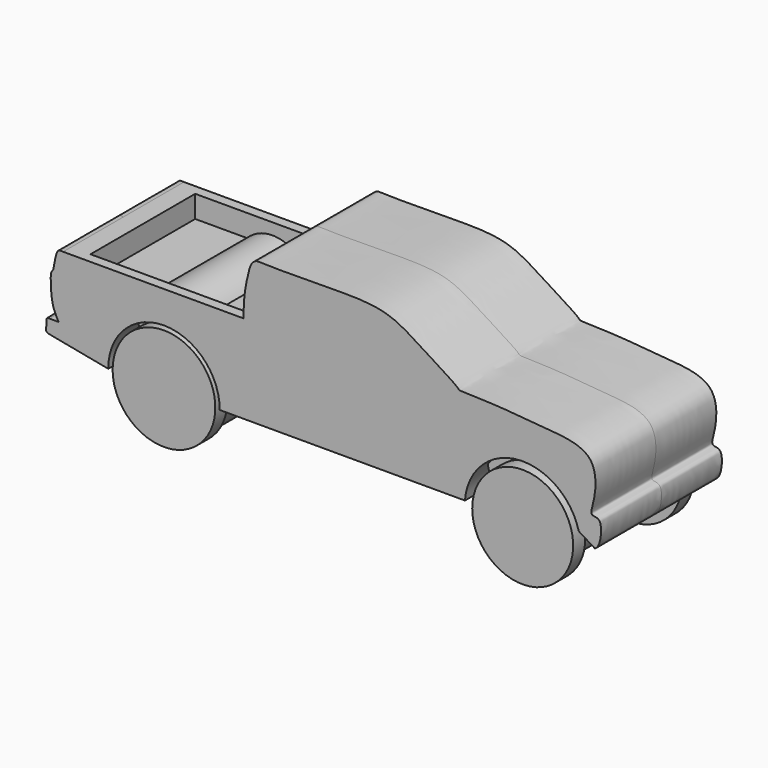
from build123d import *

# Parameters (mm, degrees)
F1_DEPTH  = 19.05
F2_W      = 40.64
F2_H      = 33.02
F3_DEPTH  = 5.588
F4_R      = 12.9540001242
F5_DEPTH  = 3.81
F4_R_2    = 12.7302206493
F9_R      = 9.0231683156
F10_DEPTH = 30.988
F11_R     = 11.353288786
F12_DEPTH = 30.988
F13_R     = 11.9558866418
F14_DEPTH = 32.258
F15_R     = 6.4554552036
F16_DEPTH = 30.734


with BuildPart() as f1:
    # F0 (on Front) → F1 (new body, symmetric)
    with BuildSketch(Plane.XZ):
        with BuildLine():
            add(Edge.make_bspline(
                [(-69.2842155695, -1.5603305073), (-69.5350025172, -1.5399307664), (-70.1964658552, -1.526121286), (-69.9018841173, -3.0286902092), (-70.3645967063, -4.8077768479), (-69.5958865333, -4.978686168), (-69.2788809538, -5.04994113)],
                knots=[0, 0, 0, 0, 0.1954252336, 0.4695328217, 0.7775236757, 1, 1, 1, 1], degree=3))
            Line((-69.2788809538, -5.04994113), (-54.4446744025, -7.8905327246))
            ThreePointArc((-54.4446744025, -7.8905327246), (-40.3995271772, 6.3133119394), (-26.354379952, -7.8905327246))
            Line((-26.354379952, -7.8905327246), (35.5073921382, -7.8905327246))
            ThreePointArc((35.5073921382, -7.8905327246), (48.7999211019, 5.5232241619), (64.2289370298, -5.3655621596))
            Line((64.2289370298, -5.3655621596), (68.332016468, -7.8905327246))
            add(Edge.make_bspline(
                [(68.332016468, -7.8905327246), (68.7067913051, -7.5679449616), (69.714492426, -6.7005653561), (70.3172984159, -0.4392585426), (66.7802927419, -1.0958089063), (68.4028013282, 2.9762612334), (69.2917253521, 14.2725497335), (53.5065140597, 14.7113305441), (43.8771565321, 16.0310681315), (33.8781446405, 15.9310273294), (33.9330328582, 16.6675611215), (26.0002542616, 21.5508658082), (18.2176068002, 26.7807544456), (11.4548434095, 28.1451041805), (3.6587892983, 28.3191044585), (-14.7558362833, 27.9741795524), (-17.1668552051, 28.3644164723), (-18.5859335818, 27.0949449022), (-19.2248198393, 24.36459907), (-20.2441867929, 19.8982618034), (-20.3211424661, 16.2882279072), (-20.3614756465, 14.3961757421)],
                knots=[0, 0, 0, 0, 0.0298592954, 0.0802861944, 0.110508584, 0.1504361757, 0.217563582, 0.2973555397, 0.3741757692, 0.438561904, 0.4519709004, 0.5165255825, 0.5881373031, 0.6432617714, 0.7085227769, 0.8031750452, 0.8361448558, 0.8632792375, 0.8998543586, 0.9475127428, 1, 1, 1, 1], degree=3))
            Line((-20.3614756465, 14.3961757421), (-65.8321008086, 14.3961757421))
            add(Edge.make_bspline(
                [(-65.8321008086, 14.3961757421), (-66.1119049823, 14.4054631172), (-66.6227405068, 14.4224189798), (-67.2879149417, 14.2751954831), (-67.9931529597, 11.9924706508), (-68.1930622811, 9.4607186493), (-69.0930767314, 9.0286087442), (-68.9238735496, 4.2425680846), (-68.3896505368, 1.0708895061), (-67.4304833389, -0.7146991208), (-66.9762343168, -1.5603305073)],
                knots=[0, 0, 0, 0, 0.0788218688, 0.1439042534, 0.2790854206, 0.4187108143, 0.4966559878, 0.6831908786, 0.8499633496, 1, 1, 1, 1], degree=3))
            Line((-66.9762343168, -1.5603305073), (-69.2842155695, -1.5603305073))
        make_face()
    extrude(amount=F1_DEPTH, both=True)

    # F2 (on face) → F3 (cut)
    with BuildSketch(Plane.XY.offset(14.3961757421)):
        with Locations((-40.6465960781, 0)):
            Rectangle(F2_W, F2_H)
    extrude(amount=-F3_DEPTH, mode=Mode.SUBTRACT)



with BuildPart() as f5:
    # F4 (on face) → F5 (new body)
    with BuildSketch(Plane(origin=(0, 19.05, 0), x_dir=(-1, 0, 0), z_dir=(0, 1, 0))):
        with Locations((40.3995271772, -7.7327218372)):
            Circle(F4_R)
    extrude(amount=-F5_DEPTH)


with BuildPart() as f5b:
    # F4 (on face) → F5, piece 2 (new body)
    with BuildSketch(Plane(origin=(0, 19.05, 0), x_dir=(-1, 0, 0), z_dir=(0, 1, 0))):
        with Locations((-50.0800661584, -9.0384282465)):
            Circle(F4_R_2)
    extrude(amount=-F5_DEPTH)


with BuildPart() as f6_1:
    # F6: instance of F5
    add(f5.part.mirror(Plane.XZ))


with BuildPart() as f6_2:
    # F6: instance of F5b
    add(f5b.part.mirror(Plane.XZ))


with BuildPart() as f1_1:
    add(f1.part)

    add(f5.part)  # F10 merges F5

    add(f6_1.part)  # F10 merges F6_1
    # F9 (on face) → F10 (join)
    with BuildSketch(Plane.XZ.offset(-15.24)):
        with Locations((-40.4575429857, 3.333261935)):
            Circle(F9_R)
    extrude(amount=F10_DEPTH)


    add(f5b.part)  # F12 merges F5b

    add(f6_2.part)  # F12 merges F6_2
    # F11 (on face) → F12 (join)
    with BuildSketch(Plane(origin=(0, -15.24, 0), x_dir=(-1, 0, 0), z_dir=(0, 1, 0))):
        with Locations((-49.4373105466, 1.3395160204)):
            Circle(F11_R)
    extrude(amount=F12_DEPTH)

    # F13 (on face) → F14 (join)
    with BuildSketch(Plane(origin=(0, -15.24, 0), x_dir=(-1, 0, 0), z_dir=(0, 1, 0))):
        with Locations((40.3995271772, -7.7327218372)):
            Circle(F13_R)
    extrude(amount=F14_DEPTH)

    # F15 (on face) → F16 (join)
    with BuildSketch(Plane(origin=(0, -15.24, 0), x_dir=(-1, 0, 0), z_dir=(0, 1, 0))):
        with Locations((-50.299461931, -13.3715048432)):
            Circle(F15_R)
    extrude(amount=F16_DEPTH)


solid = f1_1.part
